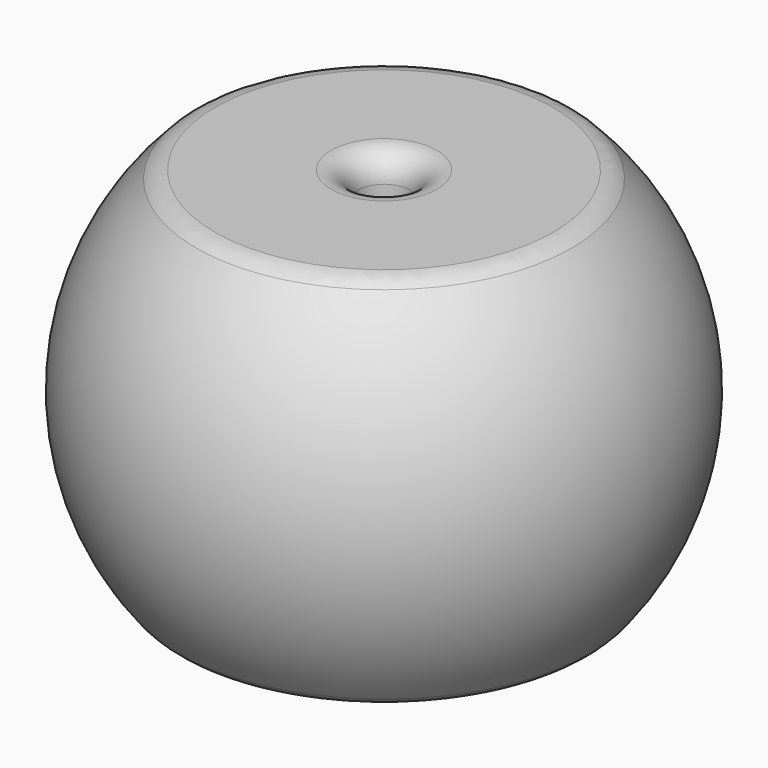
from build123d import *

# Parameters (mm, degrees)
F2_W     = 100
F2_H     = 20
F3_DEPTH = 40
F6_R     = 5
F7_DEPTH = 71.0088039765
F8_R     = 5
F9_R     = 5


with BuildPart() as f1:
    # F0 (on Front) → F1 (revolve)
    with BuildSketch(Plane.XZ):
        with BuildLine():
            Line((0, 50), (0, -50))
            ThreePointArc((0, -50), (50, 0), (0, 50))
        make_face()
    revolve(axis=Axis((0, 0, -1.8287375569), (0, 0, -1)))

    # F2 (on Front) → F3 (cut, symmetric)
    with BuildSketch(Plane.XZ):
        with Locations((0, 46.6328039765)):
            Rectangle(F2_W, F2_H)
    extrude(amount=F3_DEPTH, both=True, mode=Mode.SUBTRACT)

    # F4 (on Front) → F5 (revolve, cut)
    with BuildSketch(Plane.XZ):
        with BuildLine():
            Line((0, -25), (0, -175))
            ThreePointArc((0, -175), (75, -100), (0, -25))
        make_face()
    revolve(axis=Axis((0, 0, -99.9178830534), (0, 0, -1)), mode=Mode.SUBTRACT)

    # F6 (on face) → F7 (cut, through all)
    with BuildSketch(Plane.XY.offset(36.6328039765)):
        Circle(F6_R)
    extrude(amount=-F7_DEPTH, mode=Mode.SUBTRACT)

    # F8
    f8_edges = [f1.edges().sort_by_distance(p)[0] for p in [
        (-34.029953, 0, 36.632804),
    ]]
    fillet(f8_edges, radius=F8_R)

    # F9
    f9_edges = [f1.edges().sort_by_distance(p)[0] for p in [
        (-5, 0, 36.632804),
        (-36.309219, 0, -34.375),
        (-5, 0, -25.166852),
    ]]
    fillet(f9_edges, radius=F9_R)


solid = f1.part
